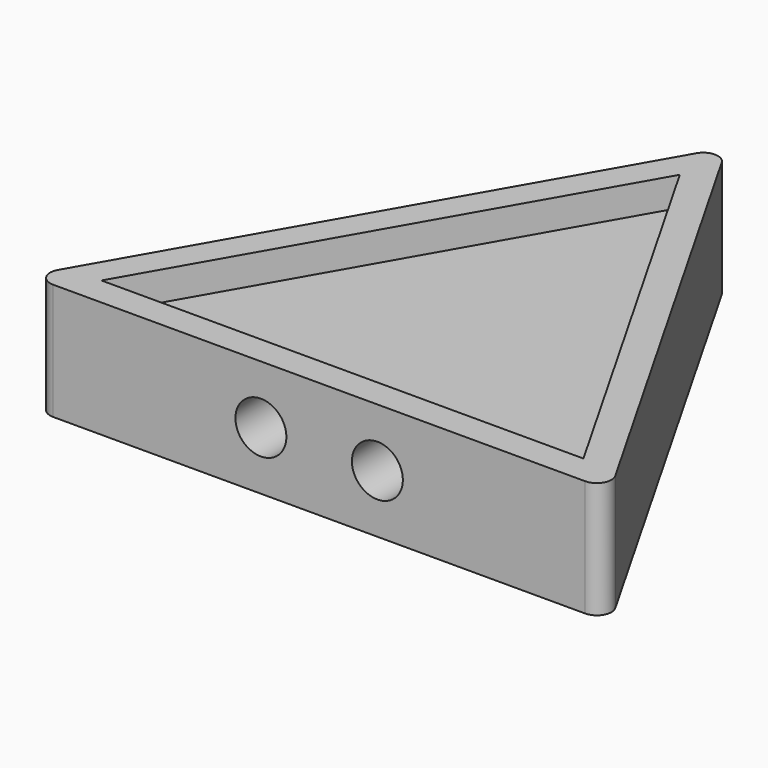
from build123d import *

# Parameters (mm, degrees)
F1_DEPTH = 8
F3_DEPTH = 2
F5_D     = 3.5
F5_DEPTH = 8
F5_TIP   = 1.0515060833
F6_R     = 1


with BuildPart() as f1:
    # F0 (on Top) → F1 (new body)
    with BuildSketch(Plane.XY):
        Polygon((0, 35), (-20, 0), (20, 0), align=None)
    extrude(amount=F1_DEPTH)

    # F2 (on face) → F3 (cut)
    with BuildSketch(Plane.XY.offset(8)):
        Polygon((0, 30.9688711259), (-16.5536406433, 2), (16.5536406433, 2), align=None)
    extrude(amount=-F3_DEPTH, mode=Mode.SUBTRACT)

    # F5
    with Locations(Plane.XZ):
        with Locations((-4, 4), (4, 4)):
            Hole(F5_D / 2, depth=F5_DEPTH)
            with Locations((0, 0, -(F5_DEPTH + F5_TIP / 2))):  # 118° drill point
                Cone(0, F5_D / 2, F5_TIP, mode=Mode.SUBTRACT)

    # F6
    f6_edges = [f1.edges().sort_by_distance(p)[0] for p in [
        (0, 35, 4),
        (-20, 0, 4),
        (20, 0, 4),
    ]]
    fillet(f6_edges, radius=F6_R)


solid = f1.part
